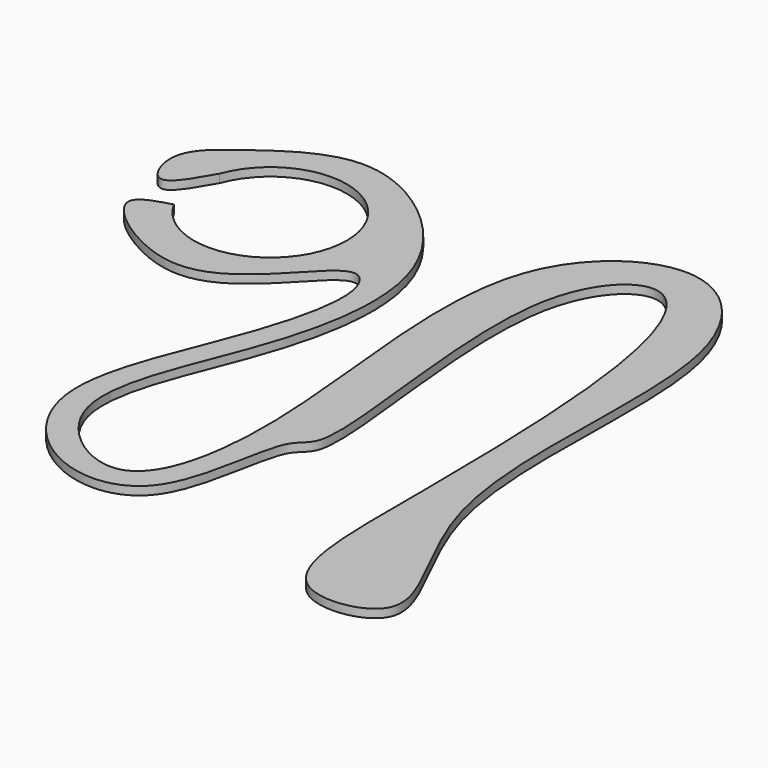
from build123d import *

# Parameters (mm, degrees)
F1_DEPTH = 1.5875


# Not quite as in the source:
# - a length typed as a fraction of an inch, garbled in the dataset ("3 / 203.2 mm" for 3/8 in), is restored


with BuildPart() as f1:
    # F0 (on Top) → F1 (new body)
    with BuildSketch(Plane.XY):
        with BuildLine():
            ThreePointArc((-18.608746289, 0), (-2.4595895568, 9.2783086346), (9.5021404255, -4.9975202419))
            ThreePointArc((9.5021404255, -4.9975202419), (-1.4152013236, -19.0476929806), (-17.7270798605, -11.9400686622))
            add(Edge.make_bspline(
                [(-18.608746289, 0), (-20.6008752956, -3.5392629392), (-24.3994951009, -10.2879796398), (-29.4789118417, 1.6089307038), (-19.4725874636, 9.082875952), (-1.9401169295, 21.3458072527), (28.7657489575, -2.8812578451), (22.724596984, -39.4806883927), (5.3015621577, -71.4294075986), (33.2879834228, -91.2116263832), (40.9325621845, -53.8672768485), (27.1101155419, 4.6221548292), (57.181168727, 24.7690532718), (80.2861230411, -0.6652403922), (67.4904349299, -61.0109872062), (96.9820223546, -94.5949025135), (68.256536538, -99.4045691849), (68.5324581278, -63.0486376972), (68.0493101716, -5.0448359229), (55.7821129266, 16.3342746577), (37.4316076141, -1.383775697), (50.5027340937, -59.0970193916), (41.2543268385, -59.7043194343), (40.5742929776, -88.2359790705), (18.8361103554, -89.2006431613), (2.2858573621, -68.9108404505), (16.6012702608, -40.0733003482), (22.2309975217, -17.7767843439), (16.4540295868, -9.7940538912), (7.6543772717, -21.106075767), (-6.2436408032, -31.2373221562), (-28.6704292793, -15.0166785816), (-20.683376113, -12.7706382317), (-17.7270798605, -11.9400686622)],
                knots=[0, 0, 0, 0, 0.0202120082, 0.0385345536, 0.0614873508, 0.0908417798, 0.1286688515, 0.1692207206, 0.2082247853, 0.238124031, 0.273733165, 0.3266485148, 0.3600750772, 0.3938425147, 0.4473761966, 0.4861703598, 0.5109443818, 0.548325465, 0.6021644918, 0.6299007231, 0.6579416514, 0.7081964032, 0.7241723861, 0.7569253665, 0.7839919014, 0.8153906941, 0.8533535119, 0.88566615, 0.901556701, 0.9246185684, 0.9523951989, 0.9822214502, 1, 1, 1, 1], degree=3))
        make_face()
    extrude(amount=F1_DEPTH)


solid = f1.part
